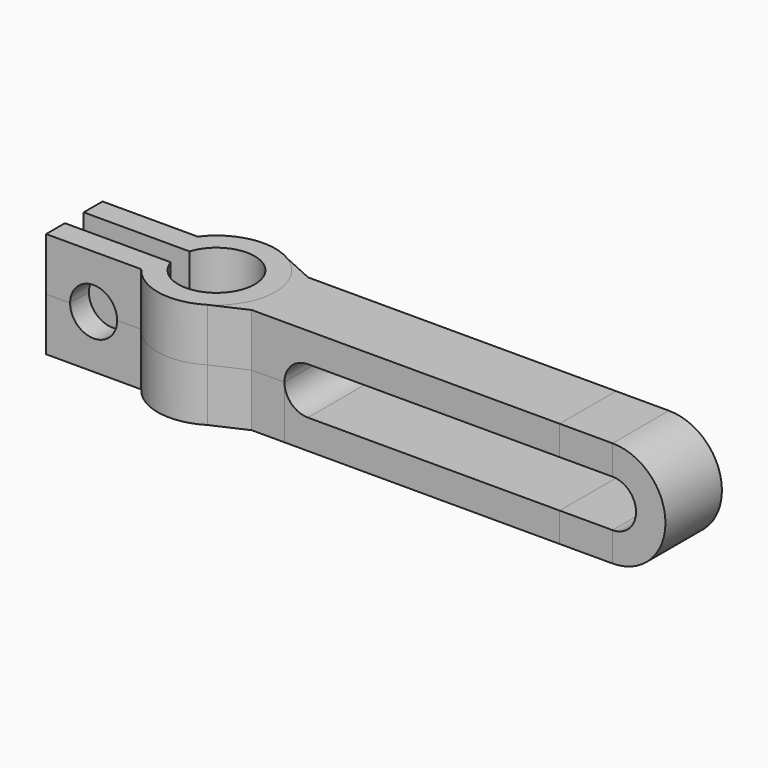
from build123d import *

# Parameters (mm, degrees)
F1_DEPTH  = 9
F2_DEPTH  = 9
F4_DEPTH  = 9
F5_DEPTH  = 9
F6_DEPTH  = 9
F8_D      = 8
F8_2_D    = 8
F3_W      = 42.8
F3_H      = 4
F9_DEPTH  = 25
F10_DEPTH = 12
F11_DEPTH = 12
F12_DEPTH = 12


# Not quite as in the source:
# - a feature names something its author has since deleted; it is built from what else it names


with BuildPart() as f1:
    # F0 (on Top) → F1 (new body)
    with BuildSketch(Plane.XY):
        with BuildLine():
            ThreePointArc((5.2753381173, -8.4953403551), (10, 0), (5.2753381173, 8.4953403551))
            ThreePointArc((5.2753381173, 8.4953403551), (-1.8473295498, 9.8278875418), (-8, 6))
            Line((-8, 6), (-24.1746007293, 6))
            Line((-24.1746007293, 6), (-24.1746007293, 2))
            Line((-24.1746007293, 2), (-8.1069414701, 2))
            Line((-8.1069414701, 2), (-6.1846584384, 2))
            ThreePointArc((-6.1846584384, 2), (6.5, 0), (-6.1846584384, -2))
            Line((-6.1846584384, -2), (-8.1069414701, -2))
            Line((-8.1069414701, -2), (-24.1746007293, -2))
            Line((-24.1746007293, -2), (-24.1746007293, -6))
            Line((-24.1746007293, -6), (-8, -6))
            ThreePointArc((-8, -6), (-1.8473295498, -9.8278875418), (5.2753381173, -8.4953403551))
        make_face()
    extrude(amount=F1_DEPTH)

    # F8 (through all)
    with Locations(Plane.XZ.offset(6)):
        with Locations((-16.0873003646, 0)):
            Hole(F8_D / 2)


with BuildPart() as f2:
    # F0 (on Top) → F2 (new body)
    with BuildSketch(Plane.XY):
        Polygon((63.15, 0), (16.35, 0), (16.35, -6), (62.2006830499, -6), (63.15, -6), (63.15, -5.0506830499), (63.15, -3.4493169501), (63.15, -2.5), align=None)
        Polygon((16.35, 6), (16.35, 0), (63.15, 0), (63.15, 2.5), (63.15, 3.4493169501), (63.15, 5.0506830499), (63.15, 6), (62.2006830499, 6), align=None)
    extrude(amount=F2_DEPTH)

    # F0 (on Top) → F4 (join)
    with BuildSketch(Plane.XY):
        with BuildLine():
            Line((16.35, -6), (16.35, 0))
            Line((16.35, 0), (16.35, 6))
            Line((16.35, 6), (10.7945588145, 6))
            Line((10.7945588145, 6), (5.2753381173, 8.4953403551))
            ThreePointArc((5.2753381173, 8.4953403551), (10, 0), (5.2753381173, -8.4953403551))
            Line((5.2753381173, -8.4953403551), (10.7945588145, -6))
            Line((10.7945588145, -6), (16.35, -6))
        make_face()
    extrude(amount=F4_DEPTH)

    # F3 (on face) → F9 (cut)
    with BuildSketch(Plane(origin=(0, 6, 0), x_dir=(-1, 0, 0), z_dir=(0, 1, 0))):
        with Locations((-41.75, 2)):
            Rectangle(F3_W, F3_H)
        Polygon((-20.35, 0), (-63.15, 0), (-63.15, -4), (-42.4068458378, -4), (-20.35, -4), align=None)
        with BuildLine():
            Line((-16.35, 0), (-20.35, 0))
            Line((-20.35, 0), (-20.35, -4))
            ThreePointArc((-20.35, -4), (-17.5215728753, -2.8284271247), (-16.35, 0))
        make_face()
        with BuildLine():
            Line((-20.35, 4), (-20.35, 0))
            Line((-20.35, 0), (-16.35, 0))
            ThreePointArc((-16.35, 0), (-17.5215728753, 2.8284271247), (-20.35, 4))
        make_face()
        with BuildLine():
            Line((-68.15, 0), (-63.15, 0))
            ThreePointArc((-63.15, 0), (-63.3875711206, 2.0542249469), (-64.0877422517, 4))
            Line((-64.0877422517, 4), (-72.15, 4))
            ThreePointArc((-72.15, 4), (-69.3215728753, 2.8284271247), (-68.15, 0))
        make_face()
        with BuildLine():
            ThreePointArc((-64.0877422517, -4), (-63.3875711206, -2.0542249469), (-63.15, 0))
            Line((-63.15, 0), (-68.15, 0))
            ThreePointArc((-68.15, 0), (-69.3215728753, -2.8284271247), (-72.15, -4))
            Line((-72.15, -4), (-64.0877422517, -4))
        make_face()
        with BuildLine():
            ThreePointArc((-64.0877422517, 4), (-63.3875711206, 2.0542249469), (-63.15, 0))
            Line((-63.15, 0), (-63.15, 4))
            Line((-63.15, 4), (-64.0877422517, 4))
        make_face()
        with BuildLine():
            Line((-63.15, -4), (-63.15, 0))
            ThreePointArc((-63.15, 0), (-63.3875711206, -2.0542249469), (-64.0877422517, -4))
            Line((-64.0877422517, -4), (-63.15, -4))
        make_face()
        with BuildLine():
            Line((-72.15, 0), (-68.15, 0))
            ThreePointArc((-68.15, 0), (-69.3215728753, 2.8284271247), (-72.15, 4))
            Line((-72.15, 4), (-72.15, 0))
        make_face()
        with BuildLine():
            ThreePointArc((-72.15, -4), (-69.3215728753, -2.8284271247), (-68.15, 0))
            Line((-68.15, 0), (-72.15, 0))
            Line((-72.15, 0), (-72.15, -4))
        make_face()
        with BuildLine():
            Line((-72.15, -4), (-72.15, 0))
            Line((-72.15, 0), (-72.15, 4))
            ThreePointArc((-72.15, 4), (-76.15, 0), (-72.15, -4))
        make_face()
    extrude(amount=-F9_DEPTH, mode=Mode.SUBTRACT)


with BuildPart() as f5:
    # F0 (on Top) → F5 (new body)
    with BuildSketch(Plane.XY):
        with BuildLine():
            Line((16.35, -6), (16.35, 0))
            Line((16.35, 0), (16.35, 6))
            Line((16.35, 6), (10.7945588145, 6))
            Line((10.7945588145, 6), (5.2753381173, 8.4953403551))
            ThreePointArc((5.2753381173, 8.4953403551), (10, 0), (5.2753381173, -8.4953403551))
            Line((5.2753381173, -8.4953403551), (10.7945588145, -6))
            Line((10.7945588145, -6), (16.35, -6))
        make_face()
    extrude(amount=-F5_DEPTH)


with BuildPart() as f6:
    # F0 (on Top) → F6 (new body)
    with BuildSketch(Plane.XY):
        with BuildLine():
            ThreePointArc((5.2753381173, -8.4953403551), (10, 0), (5.2753381173, 8.4953403551))
            ThreePointArc((5.2753381173, 8.4953403551), (-1.8473295498, 9.8278875418), (-8, 6))
            Line((-8, 6), (-24.1746007293, 6))
            Line((-24.1746007293, 6), (-24.1746007293, 2))
            Line((-24.1746007293, 2), (-8.1069414701, 2))
            Line((-8.1069414701, 2), (-6.1846584384, 2))
            ThreePointArc((-6.1846584384, 2), (6.5, 0), (-6.1846584384, -2))
            Line((-6.1846584384, -2), (-8.1069414701, -2))
            Line((-8.1069414701, -2), (-24.1746007293, -2))
            Line((-24.1746007293, -2), (-24.1746007293, -6))
            Line((-24.1746007293, -6), (-8, -6))
            ThreePointArc((-8, -6), (-1.8473295498, -9.8278875418), (5.2753381173, -8.4953403551))
        make_face()
    extrude(amount=-F6_DEPTH)

    # F8#2 (through all)
    with Locations(Plane.XZ.offset(6)):
        with Locations((-16.0873003646, 0)):
            Hole(F8_2_D / 2)


with BuildPart() as f10:
    # F3 (on face) → F10 (new body)
    with BuildSketch(Plane(origin=(0, 6, 0), x_dir=(-1, 0, 0), z_dir=(0, 1, 0))):
        with BuildLine():
            ThreePointArc((-72.15, 9), (-67.4065835097, 7.6485292704), (-64.0877422517, 4))
            Line((-64.0877422517, 4), (-63.15, 4))
            Line((-63.15, 4), (-63.15, 9))
            Line((-63.15, 9), (-72.15, 9))
        make_face()
        with BuildLine():
            Line((-72.15, 4), (-64.0877422517, 4))
            ThreePointArc((-64.0877422517, 4), (-67.4065835097, 7.6485292704), (-72.15, 9))
            Line((-72.15, 9), (-72.15, 4))
        make_face()
    extrude(amount=-F10_DEPTH)


with BuildPart() as f10b:
    # F3 (on face) → F10, piece 2 (new body)
    with BuildSketch(Plane(origin=(0, 6, 0), x_dir=(-1, 0, 0), z_dir=(0, 1, 0))):
        with BuildLine():
            Line((-63.15, -4), (-64.0877422517, -4))
            ThreePointArc((-64.0877422517, -4), (-67.4065835097, -7.6485292704), (-72.15, -9))
            Line((-72.15, -9), (-63.15, -9))
            Line((-63.15, -9), (-63.15, -4))
        make_face()
        with BuildLine():
            ThreePointArc((-72.15, -9), (-67.4065835097, -7.6485292704), (-64.0877422517, -4))
            Line((-64.0877422517, -4), (-72.15, -4))
            Line((-72.15, -4), (-72.15, -9))
        make_face()
    extrude(amount=-F10_DEPTH)


with BuildPart() as f11:
    # F3 (on face) → F11 (new body)
    with BuildSketch(Plane(origin=(0, 6, 0), x_dir=(-1, 0, 0), z_dir=(0, 1, 0))):
        Polygon((-42.4068458378, -4), (-63.15, -4), (-63.15, -9), (-16.35, -9), (-16.35, -4), (-20.35, -4), align=None)
        with BuildLine():
            Line((-16.35, -4), (-16.35, 0))
            ThreePointArc((-16.35, 0), (-17.5215728753, -2.8284271247), (-20.35, -4))
            Line((-20.35, -4), (-16.35, -4))
        make_face()
    extrude(amount=-F11_DEPTH)


with BuildPart() as f12:
    # F3 (on face) → F12 (new body)
    with BuildSketch(Plane(origin=(0, 6, 0), x_dir=(-1, 0, 0), z_dir=(0, 1, 0))):
        with BuildLine():
            ThreePointArc((-72.15, -4), (-76.15, 0), (-72.15, 4))
            Line((-72.15, 4), (-72.15, 9))
            ThreePointArc((-72.15, 9), (-81.15, 0), (-72.15, -9))
            Line((-72.15, -9), (-72.15, -4))
        make_face()
    extrude(amount=-F12_DEPTH)


solid = Compound([f1.part, f2.part, f5.part, f6.part, f10.part, f10b.part, f11.part, f12.part])
